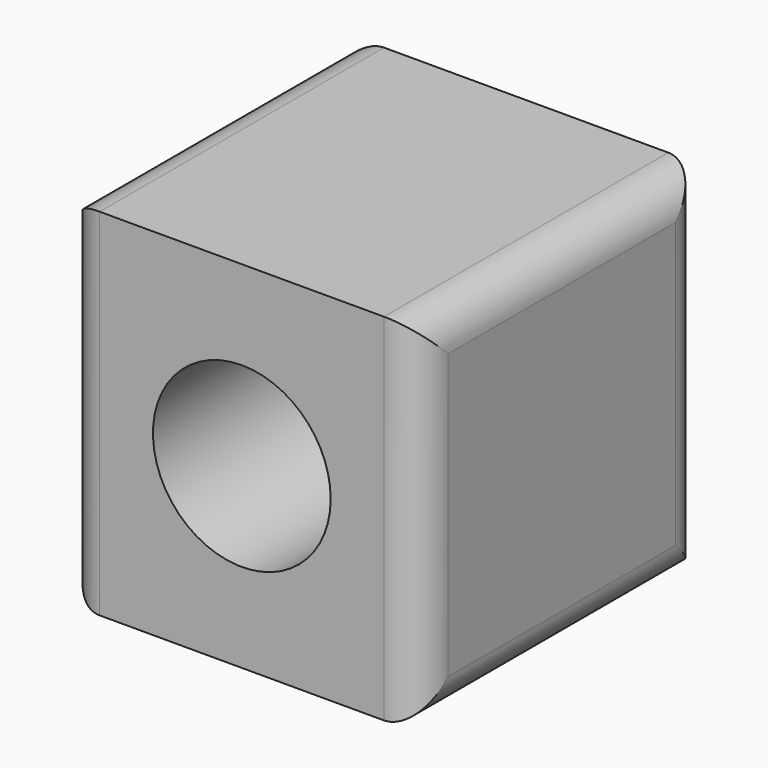
from build123d import *

# Parameters (mm, degrees)
F1_DEPTH = 50.8
F3_R     = 5.08


# Not quite as in the source:
# - the program builds the solid bodies; features that only make, move or delete a surface that nothing else refers to are left out


with BuildPart() as f1:
    # F0 (on Front) → F1 (new body)
    with BuildSketch(Plane.XZ):
        with BuildLine():
            Line((25.4, 0), (12.7, 0))
            ThreePointArc((12.7, 0), (-8.9802561211, -8.9802561211), (0, 12.7))
            Line((0, 12.7), (0, 25.4))
            Line((0, 25.4), (-25.4, 25.4))
            Line((-25.4, 25.4), (-25.4, 0))
            Line((-25.4, 0), (-25.4, -25.4))
            Line((-25.4, -25.4), (0, -25.4))
            Line((0, -25.4), (25.4, -25.4))
            Line((25.4, -25.4), (25.4, 0))
        make_face()
        with BuildLine():
            ThreePointArc((0, 12.7), (8.9802561211, 8.9802561211), (12.7, 0))
            Line((12.7, 0), (25.4, 0))
            Line((25.4, 0), (25.4, 25.4))
            Line((25.4, 25.4), (0, 25.4))
            Line((0, 25.4), (0, 12.7))
        make_face()
    extrude(amount=F1_DEPTH)

    # F3
    f3_edges = [f1.edges().sort_by_distance(p)[0] for p in [
        (-25.4, -25.4, 25.4),
        (25.4, -25.4, 25.4),
        (-25.4, -25.4, -25.4),
        (25.4, -25.4, -25.4),
        (25.4, 0, 0),
        (-25.4, 0, 0),
        (-25.4, -50.8, 0),
        (25.4, -50.8, 0),
    ]]
    fillet(f3_edges, radius=F3_R)


solid = f1.part
